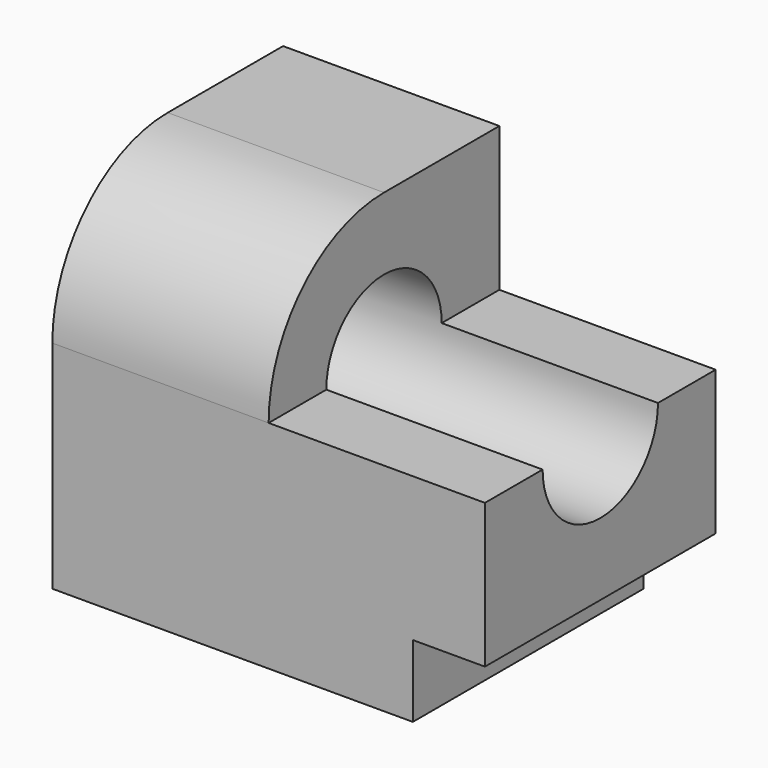
from build123d import *

# Parameters (mm, degrees)
F0_W     = 40
F0_H     = 50
F1_DEPTH = 60
F2_W     = 40
F2_H     = 20
F3_DEPTH = 30
F5_DEPTH = 60.001
F6_W     = 10
F6_H     = 10
F7_DEPTH = 40.001
F8_R     = 20


with BuildPart() as f1:
    # F0 (on Right) → F1 (new body)
    with BuildSketch(Plane.YZ):
        with Locations((20, 25)):
            Rectangle(F0_W, F0_H)
    extrude(amount=F1_DEPTH)

    # F2 (on face) → F3 (cut)
    with BuildSketch(Plane.YZ.offset(60)):
        with Locations((20, 40)):
            Rectangle(F2_W, F2_H)
    extrude(amount=-F3_DEPTH, mode=Mode.SUBTRACT)

    # F4 (on face) → F5 (cut, through all)
    with BuildSketch(Plane.YZ.offset(60)):
        with BuildLine():
            ThreePointArc((10, 30), (20, 20), (30, 30))
            Line((30, 30), (10, 30))
        make_face()
        with BuildLine():
            Line((10, 30), (30, 30))
            ThreePointArc((30, 30), (20, 40), (10, 30))
        make_face()
    extrude(amount=-F5_DEPTH, mode=Mode.SUBTRACT)

    # F6 (on face) → F7 (cut, through all)
    with BuildSketch(Plane.XZ):
        with Locations((55, 5)):
            Rectangle(F6_W, F6_H)
    extrude(amount=-F7_DEPTH, mode=Mode.SUBTRACT)

    # F8
    f8_edges = [f1.edges().sort_by_distance(p)[0] for p in [
        (15, 0, 50),
    ]]
    fillet(f8_edges, radius=F8_R)


solid = f1.part
